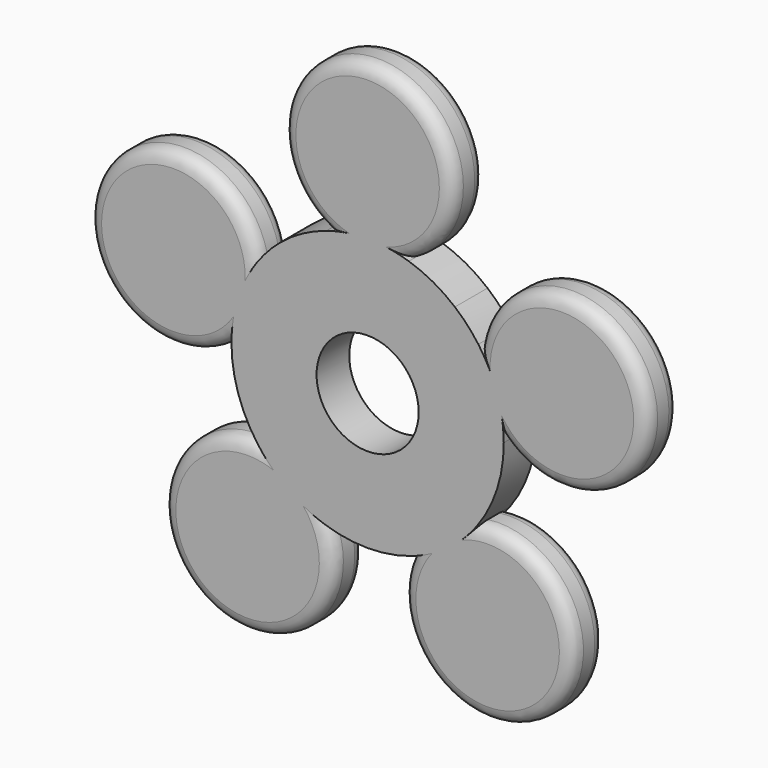
from build123d import *

# Parameters (mm, degrees)
F0_R         = 7.5
F1_DEPTH     = 6
F2_T4_ANGLE  = 348.156857
F2_S5_R      = 20
F2_T6_DEPTH  = 2104
F2_T10_ANGLE = 348.156857
F2_S11_R     = 20
F2_T12_DEPTH = 2104
F2_T16_ANGLE = 348.156857
F2_S17_R     = 20
F2_T18_DEPTH = 2094
F2_T22_ANGLE = 348.156857
F2_S23_R     = 20
F2_T24_DEPTH = 2094
F2_T28_ANGLE = 348.156857
F2_S29_R     = 20
F2_T30_DEPTH = 2087
F2_T34_ANGLE = 348.156857
F2_S35_R     = 20
F2_T36_DEPTH = 2087
F2_T40_ANGLE = 348.156857
F2_S41_R     = 20
F2_T42_DEPTH = 2106
F2_T46_ANGLE = 348.156857
F2_S47_R     = 20
F2_T48_DEPTH = 2106
F2_T52_ANGLE = 348.156857
F2_S53_R     = 20
F2_T54_DEPTH = 2074
F2_T58_ANGLE = 348.156857
F2_S59_R     = 20
F2_T60_DEPTH = 2074


# Not quite as in the source:
# - a fillet or chamfer that OpenCascade refuses, or shapes differently, is made with other operations: its cross-section is extruded or revolved along the edge and cut away or added


with BuildPart() as f1:
    # F0 (on Front) → F1 (new body)
    with BuildSketch(Plane.XZ):
        with BuildLine():
            ThreePointArc((-6.051536, 19.0625), (-9.616766, 17.536186), (-12.820394, 15.350489))
            ThreePointArc((-12.820394, 15.350489), (-14.657445, 13.607325), (-16.259487, 11.64599))
            ThreePointArc((-16.259487, 11.64599), (-40.419902, 13.133222), (-19.999542, 0.135283))
            ThreePointArc((-19.999542, 0.135283), (-19.02113, -6.18034), (-16.100452, -11.864883))
            ThreePointArc((-16.100452, -11.864883), (-24.980873, -34.383222), (-6.308861, -18.97889))
            ThreePointArc((-6.308861, -18.97889), (0, -20), (6.308861, -18.97889))
            ThreePointArc((6.308861, -18.97889), (24.980873, -34.383222), (16.100452, -11.864883))
            ThreePointArc((16.100452, -11.864883), (19.02113, -6.18034), (19.999542, 0.135283))
            ThreePointArc((19.999542, 0.135283), (40.419902, 13.133222), (16.259487, 11.64599))
            ThreePointArc((16.259487, 11.64599), (14.657445, 13.607325), (12.820394, 15.350489))
            ThreePointArc((12.820394, 15.350489), (9.616766, 17.536186), (6.051536, 19.0625))
            ThreePointArc((6.051536, 19.0625), (0, 42.5), (-6.051536, 19.0625))
        make_face()
        Circle(F0_R, mode=Mode.SUBTRACT)
    extrude(amount=F1_DEPTH)

    # F2: fillet of radius 2 on 10 edges, made by hand


with BuildPart() as f2_tool2:
    # F2_s3 → F2_t4 (revolve)
    with BuildSketch(Plane(origin=(3.078496, 0, 0.319303), x_dir=(0, 1, 0), z_dir=(-0.994664, 0, -0.103167))):
        with BuildLine():
            ThreePointArc((0.0004, -19.340887), (-0.585786, -17.925708), (-2.000966, -17.339521))
            Line((-2.000966, -17.339521), (-2.000966, -17.139385))
            ThreePointArc((-2.000966, -17.139385), (-1.000483, -17.139785), (0, -17.139785))
            Line((0, -17.139785), (0.200137, -17.339921))
            ThreePointArc((0.200137, -17.339921), (0.200137, -18.340404), (0.200537, -19.340887))
            Line((0.200537, -19.340887), (0.0004, -19.340887))
        make_face()
    revolve(axis=Axis((0, 0, 30), (0, -1, 0)), revolution_arc=F2_T4_ANGLE)

    # F2_s5 → F2_t6 (cut, symmetric)
    with BuildSketch(Plane.XZ.offset(0.5)):
        Circle(F2_S5_R)
    extrude(amount=F2_T6_DEPTH, both=True, mode=Mode.SUBTRACT)


with BuildPart() as f1_1:
    add(f1.part)

    # F2_t1: cut F2_tool2
    add(f2_tool2.part, mode=Mode.SUBTRACT)


with BuildPart() as f2_tool8:
    # F2_s9 → F2_t10 (revolve)
    with BuildSketch(Plane(origin=(3.078496, 0, 0.319303), x_dir=(0, 1, 0), z_dir=(-0.994664, 0, -0.103167))):
        with BuildLine():
            ThreePointArc((-6.0004, -19.340887), (-5.414214, -17.925708), (-3.999034, -17.339521))
            Line((-3.999034, -17.339521), (-3.999034, -17.139385))
            ThreePointArc((-3.999034, -17.139385), (-4.999517, -17.139785), (-6, -17.139785))
            Line((-6, -17.139785), (-6.200137, -17.339921))
            ThreePointArc((-6.200137, -17.339921), (-6.200137, -18.340404), (-6.200537, -19.340887))
            Line((-6.200537, -19.340887), (-6.0004, -19.340887))
        make_face()
    revolve(axis=Axis((0, -6, 30), (0, -1, 0)), revolution_arc=F2_T10_ANGLE)

    # F2_s11 → F2_t12 (cut, symmetric)
    with BuildSketch(Plane.XZ.offset(5.5)):
        Circle(F2_S11_R)
    extrude(amount=F2_T12_DEPTH, both=True, mode=Mode.SUBTRACT)


with BuildPart() as f1_2:
    add(f1_1.part)

    # F2_t7: cut F2_tool8
    add(f2_tool8.part, mode=Mode.SUBTRACT)


with BuildPart() as f2_tool14:
    # F2_s15 → F2_t16 (revolve)
    with BuildSketch(Plane(origin=(0.647632, 0, 3.026494), x_dir=(0, 1, 0), z_dir=(-0.20925, 0, -0.977862))):
        with BuildLine():
            ThreePointArc((-6.0004, -19.340887), (-5.414214, -17.925708), (-3.999034, -17.339521))
            Line((-3.999034, -17.339521), (-3.999034, -17.139385))
            ThreePointArc((-3.999034, -17.139385), (-4.999517, -17.139785), (-6, -17.139785))
            Line((-6, -17.139785), (-6.200137, -17.339921))
            ThreePointArc((-6.200137, -17.339921), (-6.200137, -18.340404), (-6.200537, -19.340887))
            Line((-6.200537, -19.340887), (-6.0004, -19.340887))
        make_face()
    revolve(axis=Axis((-28.531695, -6, 9.27051), (0, -1, 0)), revolution_arc=F2_T16_ANGLE)

    # F2_s17 → F2_t18 (cut, symmetric)
    with BuildSketch(Plane.XZ.offset(5.5)):
        Circle(F2_S17_R)
    extrude(amount=F2_T18_DEPTH, both=True, mode=Mode.SUBTRACT)


with BuildPart() as f1_3:
    add(f1_2.part)

    # F2_t13: cut F2_tool14
    add(f2_tool14.part, mode=Mode.SUBTRACT)


with BuildPart() as f2_tool20:
    # F2_s21 → F2_t22 (revolve)
    with BuildSketch(Plane(origin=(0.647632, 0, 3.026494), x_dir=(0, 1, 0), z_dir=(-0.20925, 0, -0.977862))):
        with BuildLine():
            ThreePointArc((-2.000966, -17.339521), (-0.585786, -17.925708), (0.0004, -19.340887))
            Line((0.0004, -19.340887), (0.200537, -19.340887))
            ThreePointArc((0.200537, -19.340887), (0.200137, -18.340404), (0.200137, -17.339921))
            Line((0.200137, -17.339921), (0, -17.139785))
            ThreePointArc((0, -17.139785), (-1.000483, -17.139785), (-2.000966, -17.139385))
            Line((-2.000966, -17.139385), (-2.000966, -17.339521))
        make_face()
    revolve(axis=Axis((-28.531695, 0, 9.27051), (0, -1, 0)), revolution_arc=F2_T22_ANGLE)

    # F2_s23 → F2_t24 (cut, symmetric)
    with BuildSketch(Plane.XZ.offset(0.5)):
        Circle(F2_S23_R)
    extrude(amount=F2_T24_DEPTH, both=True, mode=Mode.SUBTRACT)


with BuildPart() as f1_4:
    add(f1_3.part)

    # F2_t19: cut F2_tool20
    add(f2_tool20.part, mode=Mode.SUBTRACT)


with BuildPart() as f2_tool26:
    # F2_s27 → F2_t28 (revolve)
    with BuildSketch(Plane(origin=(-2.678237, 0, 1.551173), x_dir=(0, 1, 0), z_dir=(0.86534, 0, -0.501185))):
        with BuildLine():
            ThreePointArc((-6.0004, -19.340887), (-5.414214, -17.925708), (-3.999034, -17.339521))
            Line((-3.999034, -17.339521), (-3.999034, -17.139385))
            ThreePointArc((-3.999034, -17.139385), (-4.999517, -17.139785), (-6, -17.139785))
            Line((-6, -17.139785), (-6.200137, -17.339921))
            ThreePointArc((-6.200137, -17.339921), (-6.200137, -18.340404), (-6.200537, -19.340887))
            Line((-6.200537, -19.340887), (-6.0004, -19.340887))
        make_face()
    revolve(axis=Axis((-17.633558, -6, -24.27051), (0, -1, 0)), revolution_arc=F2_T28_ANGLE)

    # F2_s29 → F2_t30 (cut, symmetric)
    with BuildSketch(Plane.XZ.offset(5.5)):
        Circle(F2_S29_R)
    extrude(amount=F2_T30_DEPTH, both=True, mode=Mode.SUBTRACT)


with BuildPart() as f1_5:
    add(f1_4.part)

    # F2_t25: cut F2_tool26
    add(f2_tool26.part, mode=Mode.SUBTRACT)


with BuildPart() as f2_tool32:
    # F2_s33 → F2_t34 (revolve)
    with BuildSketch(Plane(origin=(-2.678237, 0, 1.551173), x_dir=(0, 1, 0), z_dir=(0.86534, 0, -0.501185))):
        with BuildLine():
            ThreePointArc((-2.000966, -17.339521), (-0.585786, -17.925708), (0.0004, -19.340887))
            Line((0.0004, -19.340887), (0.200537, -19.340887))
            ThreePointArc((0.200537, -19.340887), (0.200137, -18.340404), (0.200137, -17.339921))
            Line((0.200137, -17.339921), (0, -17.139785))
            ThreePointArc((0, -17.139785), (-1.000483, -17.139785), (-2.000966, -17.139385))
            Line((-2.000966, -17.139385), (-2.000966, -17.339521))
        make_face()
    revolve(axis=Axis((-17.633558, 0, -24.27051), (0, -1, 0)), revolution_arc=F2_T34_ANGLE)

    # F2_s35 → F2_t36 (cut, symmetric)
    with BuildSketch(Plane.XZ.offset(0.5)):
        Circle(F2_S35_R)
    extrude(amount=F2_T36_DEPTH, both=True, mode=Mode.SUBTRACT)


with BuildPart() as f1_6:
    add(f1_5.part)

    # F2_t31: cut F2_tool32
    add(f2_tool32.part, mode=Mode.SUBTRACT)


with BuildPart() as f2_tool38:
    # F2_s39 → F2_t40 (revolve)
    with BuildSketch(Plane(origin=(-2.302874, 0, -2.067816), x_dir=(0, 1, 0), z_dir=(0.74406, 0, 0.668113))):
        with BuildLine():
            ThreePointArc((-6.0004, -19.340887), (-5.414214, -17.925708), (-3.999034, -17.339521))
            Line((-3.999034, -17.339521), (-3.999034, -17.139385))
            ThreePointArc((-3.999034, -17.139385), (-4.999517, -17.139785), (-6, -17.139785))
            Line((-6, -17.139785), (-6.200137, -17.339921))
            ThreePointArc((-6.200137, -17.339921), (-6.200137, -18.340404), (-6.200537, -19.340887))
            Line((-6.200537, -19.340887), (-6.0004, -19.340887))
        make_face()
    revolve(axis=Axis((17.633558, -6, -24.27051), (0, -1, 0)), revolution_arc=F2_T40_ANGLE)

    # F2_s41 → F2_t42 (cut, symmetric)
    with BuildSketch(Plane.XZ.offset(5.5)):
        Circle(F2_S41_R)
    extrude(amount=F2_T42_DEPTH, both=True, mode=Mode.SUBTRACT)


with BuildPart() as f1_7:
    add(f1_6.part)

    # F2_t37: cut F2_tool38
    add(f2_tool38.part, mode=Mode.SUBTRACT)


with BuildPart() as f2_tool44:
    # F2_s45 → F2_t46 (revolve)
    with BuildSketch(Plane(origin=(-2.302874, 0, -2.067816), x_dir=(0, 1, 0), z_dir=(0.74406, 0, 0.668113))):
        with BuildLine():
            ThreePointArc((-2.000966, -17.339521), (-0.585786, -17.925708), (0.0004, -19.340887))
            Line((0.0004, -19.340887), (0.200537, -19.340887))
            ThreePointArc((0.200537, -19.340887), (0.200137, -18.340404), (0.200137, -17.339921))
            Line((0.200137, -17.339921), (0, -17.139785))
            ThreePointArc((0, -17.139785), (-1.000483, -17.139785), (-2.000966, -17.139385))
            Line((-2.000966, -17.139385), (-2.000966, -17.339521))
        make_face()
    revolve(axis=Axis((17.633558, 0, -24.27051), (0, -1, 0)), revolution_arc=F2_T46_ANGLE)

    # F2_s47 → F2_t48 (cut, symmetric)
    with BuildSketch(Plane.XZ.offset(0.5)):
        Circle(F2_S47_R)
    extrude(amount=F2_T48_DEPTH, both=True, mode=Mode.SUBTRACT)


with BuildPart() as f1_8:
    add(f1_7.part)

    # F2_t43: cut F2_tool44
    add(f2_tool44.part, mode=Mode.SUBTRACT)


with BuildPart() as f2_tool50:
    # F2_s51 → F2_t52 (revolve)
    with BuildSketch(Plane(origin=(1.254983, 0, -2.829154), x_dir=(0, 1, 0), z_dir=(-0.405486, 0, 0.914101))):
        with BuildLine():
            ThreePointArc((-6.0004, -19.340887), (-5.414214, -17.925708), (-3.999034, -17.339521))
            Line((-3.999034, -17.339521), (-3.999034, -17.139385))
            ThreePointArc((-3.999034, -17.139385), (-4.999517, -17.139785), (-6, -17.139785))
            Line((-6, -17.139785), (-6.200137, -17.339921))
            ThreePointArc((-6.200137, -17.339921), (-6.200137, -18.340404), (-6.200537, -19.340887))
            Line((-6.200537, -19.340887), (-6.0004, -19.340887))
        make_face()
    revolve(axis=Axis((28.531695, -6, 9.27051), (0, -1, 0)), revolution_arc=F2_T52_ANGLE)

    # F2_s53 → F2_t54 (cut, symmetric)
    with BuildSketch(Plane.XZ.offset(5.5)):
        Circle(F2_S53_R)
    extrude(amount=F2_T54_DEPTH, both=True, mode=Mode.SUBTRACT)


with BuildPart() as f1_9:
    add(f1_8.part)

    # F2_t49: cut F2_tool50
    add(f2_tool50.part, mode=Mode.SUBTRACT)


with BuildPart() as f2_tool56:
    # F2_s57 → F2_t58 (revolve)
    with BuildSketch(Plane(origin=(1.254983, 0, -2.829154), x_dir=(0, 1, 0), z_dir=(-0.405486, 0, 0.914101))):
        with BuildLine():
            ThreePointArc((-2.000966, -17.339521), (-0.585786, -17.925708), (0.0004, -19.340887))
            Line((0.0004, -19.340887), (0.200537, -19.340887))
            ThreePointArc((0.200537, -19.340887), (0.200137, -18.340404), (0.200137, -17.339921))
            Line((0.200137, -17.339921), (0, -17.139785))
            ThreePointArc((0, -17.139785), (-1.000483, -17.139785), (-2.000966, -17.139385))
            Line((-2.000966, -17.139385), (-2.000966, -17.339521))
        make_face()
    revolve(axis=Axis((28.531695, 0, 9.27051), (0, -1, 0)), revolution_arc=F2_T58_ANGLE)

    # F2_s59 → F2_t60 (cut, symmetric)
    with BuildSketch(Plane.XZ.offset(0.5)):
        Circle(F2_S59_R)
    extrude(amount=F2_T60_DEPTH, both=True, mode=Mode.SUBTRACT)


with BuildPart() as f1_10:
    add(f1_9.part)

    # F2_t55: cut F2_tool56
    add(f2_tool56.part, mode=Mode.SUBTRACT)


solid = f1_10.part
